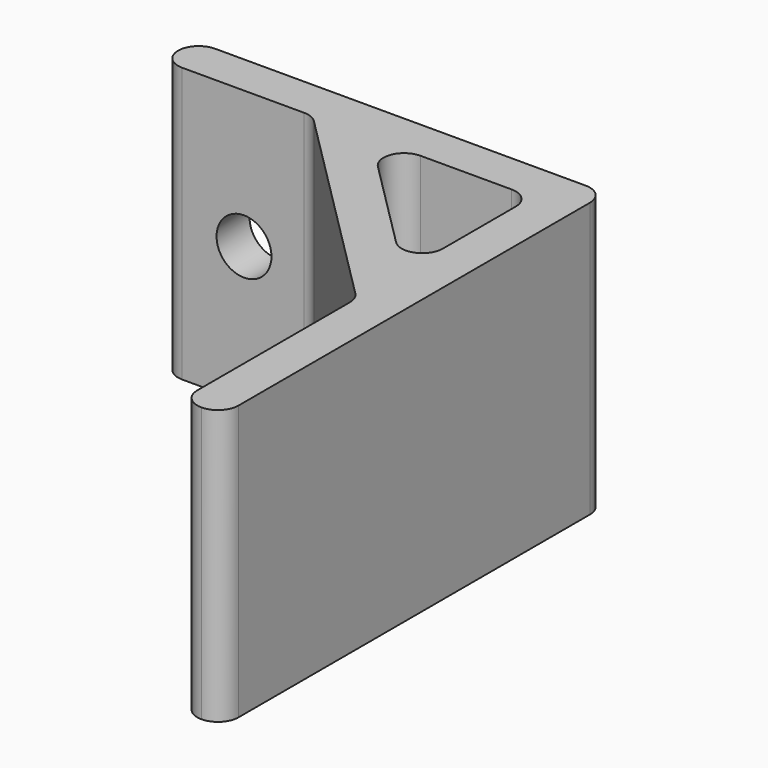
from build123d import *

# Parameters (mm, degrees)
F1_DEPTH = 20
F3_R     = 1.49999
F2_R     = 2
F4_DEPTH = 3


# Not quite as in the source:
# - a fillet or chamfer is up to 0.001 mm smaller than in the source, because OpenCascade refuses the exact size


with BuildPart() as f1:
    # F0 (on Top) → F1 (new body)
    with BuildSketch(Plane.XY):
        Polygon((11, 11), (-19, 11), (-19, 8), (-8, 8), (-3.7573593129, 8), (8, 8), (8, -3.7573593129), (8, -8), (8, -24), (11, -24), align=None)
        Polygon((-3.7573593129, 8), (-8, 8), (8, -8), (8, -3.7573593129), align=None)
    extrude(amount=F1_DEPTH)

    # F3 (radius 1.5 in the source; OpenCascade refuses exactly that, so slightly less here)
    f3_edges = [f1.edges().sort_by_distance(p)[0] for p in [
        (-19, 8, 10),
        (-19, 11, 10),
        (-8, 8, 10),
        (8, -24, 10),
        (11, -24, 10),
        (8, -8, 10),
        (8, 8, 10),
        (11, 11, 10),
        (-3.757359, 8, 10),
        (8, -3.757359, 10),
    ]]
    fillet(f3_edges, radius=F3_R)

    # F2 (on face) → F4 (cut, through all)
    with BuildSketch(Plane.XZ.offset(-8)):
        with Locations((-13, 10)):
            Circle(F2_R)
    extrude(amount=-F4_DEPTH, mode=Mode.SUBTRACT)


solid = f1.part
